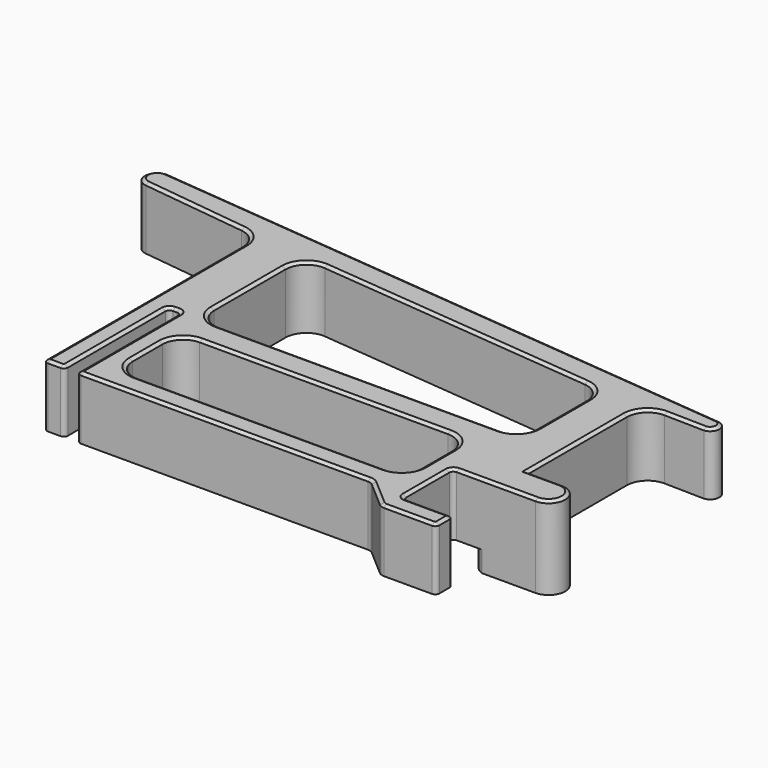
from build123d import *

# Parameters (mm, degrees)
F1_DEPTH      = 19.05
F2_T1_DEPTH   = 75.2234896329
F2_T3_DEPTH   = 3.81
F2_T5_DEPTH   = 37.3962257746
F2_T7_DEPTH   = 1.27
F2_T9_DEPTH   = 88.0190491883
F2_T11_DEPTH  = 10.8349024574
F2_T13_DEPTH  = 14.7622946385
F2_T15_DEPTH  = 3.81
F2_T17_DEPTH  = 12.6952033794
F2_T19_DEPTH  = 16.5052033794
F2_T21_DEPTH  = 24.13
F2_T23_DEPTH  = 10.16
F2_T25_DEPTH  = 35.52184429
F2_T28_ANGLE  = 83.061791683
F2_T30_ANGLE  = 90
F2_T32_ANGLE  = 90
F2_T34_ANGLE  = 90
F2_T36_ANGLE  = 90
F2_T38_ANGLE  = 90
F2_T40_ANGLE  = 40.847550521
F2_T42_ANGLE  = 40.8475505209
F2_T44_ANGLE  = 90
F2_T46_ANGLE  = 90
F2_T48_ANGLE  = 90
F2_T50_ANGLE  = 90
F2_T52_ANGLE  = 180
F2_T53_DEPTH  = 15.1008716715
F2_T58_DEPTH  = 41.6145620658
F2_T63_DEPTH  = 41.6145620658
F2_T69_DEPTH  = 41.6145620658
F2_T73_ANGLE  = 91.1976782387
F2_T74_DEPTH  = 183.8355440501
F2_T77_ANGLE  = 180.467792794
F2_T79_ANGLE  = 176.997776884
F2_T80_DEPTH  = 76.2
F2_T82_DEPTH  = 11.4254270077
F2_T85_ANGLE  = 90
F2_T87_ANGLE  = 90
F2_T89_ANGLE  = 90
F2_T91_ANGLE  = 90
F2_T92_DEPTH  = 19.192433885
F2_T94_DEPTH  = 86.36
F2_T96_DEPTH  = 27.4006934119
F2_T98_DEPTH  = 86.7492082065
F2_T101_ANGLE = 84.5705182986
F2_T103_ANGLE = 90
F2_T105_ANGLE = 90
F2_T107_ANGLE = 95.4294817014
F4_DEPTH      = 6.35


# Not quite as in the source:
# - a fillet or chamfer that OpenCascade refuses, or shapes differently, is made with other operations: its cross-section is extruded or revolved along the edge and cut away or added


with BuildPart() as f1:
    # F0 (on Top) → F1 (new body)
    with BuildSketch(Plane.XY):
        with BuildLine():
            Line((-61.3219774175, -39.9362257746), (-47.7384642892, -39.9362257746))
            Line((-47.7384642892, -39.9362257746), (26.6970717708, -39.9362257746))
            ThreePointArc((26.6970717708, -39.9362257746), (27.5834325804, -40.0958971176), (28.3583552632, -40.5548363924))
            Line((28.3583552632, -40.5548363924), (36.5544444517, -47.6413893822))
            ThreePointArc((36.5544444517, -47.6413893822), (37.3293671345, -48.100328657), (38.215727944, -48.26))
            Line((38.215727944, -48.26), (52.9780225825, -48.26))
            ThreePointArc((52.9780225825, -48.26), (53.8760481946, -47.8880256121), (54.2480225825, -46.99))
            Line((54.2480225825, -46.99), (54.2480225825, -43.18))
            ThreePointArc((54.2480225825, -43.18), (53.8760481946, -42.2819743879), (52.9780225825, -41.91))
            Line((52.9780225825, -41.91), (40.2828192031, -41.91))
            ThreePointArc((40.2828192031, -41.91), (39.3814018681, -41.5366207145), (39.0080225825, -40.6352033794))
            Line((39.0080225825, -40.6352033794), (39.0080225825, -24.13))
            ThreePointArc((39.0080225825, -24.13), (39.3799969704, -23.2319743879), (40.2780225825, -22.86))
            Line((40.2780225825, -22.86), (56.7928192031, -22.86))
            Line((56.7928192031, -22.86), (64.4080225825, -22.86))
            ThreePointArc((64.4080225825, -22.86), (69.4880225825, -17.78), (64.4080225825, -12.7))
            Line((64.4080225825, -12.7), (54.2480225825, -12.7))
            Line((54.2480225825, -12.7), (54.2480225825, 0))
            Line((54.2480225825, 0), (54.2480225825, 24.9692976817))
            ThreePointArc((54.2480225825, 24.9692976817), (56.1550684482, 29.5061091787), (60.730749688, 31.3179104053))
            Line((60.730749688, 31.3179104053), (72.9835318038, 31.0617479373))
            ThreePointArc((72.9835318038, 31.0617479373), (75.4911679584, 33.8910968404), (72.9375934671, 36.6790551646))
            Line((72.9375934671, 36.6790551646), (-110.0535898834, 54.2783185637))
            ThreePointArc((-110.0535898834, 54.2783185637), (-114.147959014, 50.9024071856), (-110.772047636, 46.808038055))
            Line((-110.772047636, 46.808038055), (-78.3349047634, 42.8607628504))
            ThreePointArc((-78.3349047634, 42.8607628504), (-74.3483781836, 40.7674650795), (-72.7519774175, 36.5572638583))
            Line((-72.7519774175, 36.5572638583), (-72.7519774175, 0))
            Line((-72.7519774175, 0), (-72.7519774175, -24.13))
            Line((-72.7519774175, -24.13), (-72.7519774175, -38.6662257746))
            ThreePointArc((-72.7519774175, -38.6662257746), (-72.3800030296, -39.5642513867), (-71.4819774175, -39.9362257746))
            Line((-71.4819774175, -39.9362257746), (-67.6719774175, -39.9362257746))
            ThreePointArc((-67.6719774175, -39.9362257746), (-66.7739518054, -39.5642513867), (-66.4019774175, -38.6662257746))
            Line((-66.4019774175, -38.6662257746), (-66.4019774175, -24.13))
            Line((-66.4019774175, -24.13), (-66.4019774175, -1.27))
            ThreePointArc((-66.4019774175, -1.27), (-66.0300030296, -0.3719743879), (-65.1319774175, 0))
            Line((-65.1319774175, 0), (-63.8619774175, 0))
            ThreePointArc((-63.8619774175, 0), (-62.9639518054, -0.3719743879), (-62.5919774175, -1.27))
            Line((-62.5919774175, -1.27), (-62.5919774175, -24.13))
            Line((-62.5919774175, -24.13), (-62.5919774175, -38.6662257746))
            ThreePointArc((-62.5919774175, -38.6662257746), (-62.2200030296, -39.5642513867), (-61.3219774175, -39.9362257746))
        make_face()
        with BuildLine():
            ThreePointArc((-56.2419774175, -15.0875305593), (-54.382105478, -10.5974024988), (-49.8919774175, -8.7375305593))
            Line((-49.8919774175, -8.7375305593), (26.3080225825, -8.7375305593))
            ThreePointArc((26.3080225825, -8.7375305593), (30.7981506431, -10.5974024988), (32.6580225825, -15.0875305593))
            Line((32.6580225825, -15.0875305593), (32.6580225825, -26.512957567))
            ThreePointArc((32.6580225825, -26.512957567), (30.7981506431, -31.0030856275), (26.3080225825, -32.862957567))
            Line((26.3080225825, -32.862957567), (-49.8919774175, -32.862957567))
            ThreePointArc((-49.8919774175, -32.862957567), (-54.382105478, -31.0030856275), (-56.2419774175, -26.512957567))
            Line((-56.2419774175, -26.512957567), (-56.2419774175, -15.0875305593))
        make_face(mode=Mode.SUBTRACT)
        with BuildLine():
            ThreePointArc((35.798863202, 31.8639440329), (39.8957793841, 29.8148548653), (41.5480225825, 25.542433885))
            Line((41.5480225825, 25.542433885), (41.5480225825, 6.35))
            ThreePointArc((41.5480225825, 6.35), (39.6881506431, 1.8598719395), (35.1980225825, 0))
            Line((35.1980225825, 0), (-51.1619774175, 0))
            ThreePointArc((-51.1619774175, 0), (-55.652105478, 1.8598719395), (-57.5119774175, 6.35))
            Line((-57.5119774175, 6.35), (-57.5119774175, 33.7506934119))
            ThreePointArc((-57.5119774175, 33.7506934119), (-55.4343983978, 38.4484502135), (-50.561136798, 40.0722035598))
            Line((-50.561136798, 40.0722035598), (35.798863202, 31.8639440329))
        make_face(mode=Mode.SUBTRACT)
    extrude(amount=F1_DEPTH)

    # F2: chamfer of 0.635 x 1.0998522628 on 49 edges, made by hand

    # F2_s2 → F2_t1 (cut)
    with BuildSketch(Plane.XZ.offset(-36.5572638583)):
        with BuildLine():
            Line((-71.6140251547, 19.0719970453), (-72.7900774175, 18.3930029547))
            Line((-72.7900774175, 18.3930029547), (-72.8120744627, 18.3930029547))
            ThreePointArc((-72.8120744627, 18.3930029547), (-72.7739744627, 18.7215014774), (-72.7739744627, 19.05))
            Line((-72.7739744627, 19.05), (-72.7519774175, 19.0719970453))
            ThreePointArc((-72.7519774175, 19.0719970453), (-72.1830012861, 19.0719970453), (-71.6140251547, 19.0939940905))
            Line((-71.6140251547, 19.0939940905), (-71.6140251547, 19.0719970453))
        make_face()
    extrude(amount=F2_T1_DEPTH, mode=Mode.SUBTRACT)

    # F2_s4 → F2_t3 (cut)
    with BuildSketch(Plane.YZ.offset(-71.4819774175)):
        with BuildLine():
            Line((-38.7982735118, 19.0719970453), (-39.9743257746, 18.3930029547))
            Line((-39.9743257746, 18.3930029547), (-39.9963228198, 18.3930029547))
            ThreePointArc((-39.9963228198, 18.3930029547), (-39.9582228198, 18.7215014774), (-39.9582228198, 19.05))
            Line((-39.9582228198, 19.05), (-39.9362257746, 19.0719970453))
            ThreePointArc((-39.9362257746, 19.0719970453), (-39.3672496432, 19.0719970453), (-38.7982735118, 19.0939940905))
            Line((-38.7982735118, 19.0939940905), (-38.7982735118, 19.0719970453))
        make_face()
    extrude(amount=F2_T3_DEPTH, mode=Mode.SUBTRACT)

    # F2_s6 → F2_t5 (cut)
    with BuildSketch(Plane.XZ.offset(1.27)):
        with BuildLine():
            Line((-67.5399296803, 19.0719970453), (-66.3638774175, 18.3930029547))
            Line((-66.3638774175, 18.3930029547), (-66.3418803722, 18.3930029547))
            ThreePointArc((-66.3418803722, 18.3930029547), (-66.3799803722, 18.7215014774), (-66.3799803722, 19.05))
            Line((-66.3799803722, 19.05), (-66.4019774175, 19.0719970453))
            ThreePointArc((-66.4019774175, 19.0719970453), (-66.9709535489, 19.0719970453), (-67.5399296803, 19.0939940905))
            Line((-67.5399296803, 19.0939940905), (-67.5399296803, 19.0719970453))
        make_face()
        with BuildLine():
            Line((-61.4540251547, 19.0719970453), (-62.6300774175, 18.3930029547))
            Line((-62.6300774175, 18.3930029547), (-62.6520744627, 18.3930029547))
            ThreePointArc((-62.6520744627, 18.3930029547), (-62.6139744627, 18.7215014774), (-62.6139744627, 19.05))
            Line((-62.6139744627, 19.05), (-62.5919774175, 19.0719970453))
            ThreePointArc((-62.5919774175, 19.0719970453), (-62.0230012861, 19.0719970453), (-61.4540251547, 19.0939940905))
            Line((-61.4540251547, 19.0939940905), (-61.4540251547, 19.0719970453))
        make_face()
    extrude(amount=F2_T5_DEPTH, mode=Mode.SUBTRACT)

    # F2_s8 → F2_t7 (cut)
    with BuildSketch(Plane.YZ.offset(-65.1319774175)):
        with BuildLine():
            Line((1.1379522628, 19.0719970453), (-0.0381, 18.3930029547))
            Line((-0.0381, 18.3930029547), (-0.0600970453, 18.3930029547))
            ThreePointArc((-0.0600970453, 18.3930029547), (-0.0219970453, 18.7215014774), (-0.0219970453, 19.05))
            Line((-0.0219970453, 19.05), (0, 19.0719970453))
            ThreePointArc((0, 19.0719970453), (0.5689761314, 19.0719970453), (1.1379522628, 19.0939940905))
            Line((1.1379522628, 19.0939940905), (1.1379522628, 19.0719970453))
        make_face()
    extrude(amount=F2_T7_DEPTH, mode=Mode.SUBTRACT)

    # F2_s10 → F2_t9 (cut)
    with BuildSketch(Plane.YZ.offset(-61.3219774175)):
        with BuildLine():
            Line((-38.7982735118, 19.0719970453), (-39.9743257746, 18.3930029547))
            Line((-39.9743257746, 18.3930029547), (-39.9963228198, 18.3930029547))
            ThreePointArc((-39.9963228198, 18.3930029547), (-39.9582228198, 18.7215014774), (-39.9582228198, 19.05))
            Line((-39.9582228198, 19.05), (-39.9362257746, 19.0719970453))
            ThreePointArc((-39.9362257746, 19.0719970453), (-39.3672496432, 19.0719970453), (-38.7982735118, 19.0939940905))
            Line((-38.7982735118, 19.0939940905), (-38.7982735118, 19.0719970453))
        make_face()
    extrude(amount=F2_T9_DEPTH, mode=Mode.SUBTRACT)

    # F2_s12 → F2_t11 (cut)
    with BuildSketch(Plane(origin=(36.2920073891, -31.379018402, 0), x_dir=(0, 0, 1), z_dir=(0.7564525127, -0.654048619, 0))):
        with BuildLine():
            Line((19.0719970453, 10.9921125288), (18.3930029547, 12.1681647916))
            Line((18.3930029547, 12.1681647916), (18.3930029547, 12.1901618368))
            ThreePointArc((18.3930029547, 12.1901618368), (18.7215014774, 12.1520618368), (19.05, 12.1520618368))
            Line((19.05, 12.1520618368), (19.0719970453, 12.1300647916))
            ThreePointArc((19.0719970453, 12.1300647916), (19.0719970453, 11.5610886602), (19.0939940905, 10.9921125288))
            Line((19.0939940905, 10.9921125288), (19.0719970453, 10.9921125288))
        make_face()
    extrude(amount=F2_T11_DEPTH, mode=Mode.SUBTRACT)

    # F2_s14 → F2_t13 (cut)
    with BuildSketch(Plane.YZ.offset(38.215727944)):
        with BuildLine():
            Line((-47.1220477372, 19.0719970453), (-48.2981, 18.3930029547))
            Line((-48.2981, 18.3930029547), (-48.3200970453, 18.3930029547))
            ThreePointArc((-48.3200970453, 18.3930029547), (-48.2819970453, 18.7215014774), (-48.2819970453, 19.05))
            Line((-48.2819970453, 19.05), (-48.26, 19.0719970453))
            ThreePointArc((-48.26, 19.0719970453), (-47.6910238686, 19.0719970453), (-47.1220477372, 19.0939940905))
            Line((-47.1220477372, 19.0939940905), (-47.1220477372, 19.0719970453))
        make_face()
    extrude(amount=F2_T13_DEPTH, mode=Mode.SUBTRACT)

    # F2_s16 → F2_t15 (cut)
    with BuildSketch(Plane.XZ.offset(43.18)):
        with BuildLine():
            Line((53.1100703197, 19.0719970453), (54.2861225825, 18.3930029547))
            Line((54.2861225825, 18.3930029547), (54.3081196278, 18.3930029547))
            ThreePointArc((54.3081196278, 18.3930029547), (54.2700196278, 18.7215014774), (54.2700196278, 19.05))
            Line((54.2700196278, 19.05), (54.2480225825, 19.0719970453))
            ThreePointArc((54.2480225825, 19.0719970453), (53.6790464511, 19.0719970453), (53.1100703197, 19.0939940905))
            Line((53.1100703197, 19.0939940905), (53.1100703197, 19.0719970453))
        make_face()
    extrude(amount=F2_T15_DEPTH, mode=Mode.SUBTRACT)

    # F2_s18 → F2_t17 (cut)
    with BuildSketch(Plane.YZ.offset(40.2828192031)):
        with BuildLine():
            Line((-43.0479522628, 19.0719970453), (-41.8719, 18.3930029547))
            Line((-41.8719, 18.3930029547), (-41.8499029547, 18.3930029547))
            ThreePointArc((-41.8499029547, 18.3930029547), (-41.8880029547, 18.7215014774), (-41.8880029547, 19.05))
            Line((-41.8880029547, 19.05), (-41.91, 19.0719970453))
            ThreePointArc((-41.91, 19.0719970453), (-42.4789761314, 19.0719970453), (-43.0479522628, 19.0939940905))
            Line((-43.0479522628, 19.0939940905), (-43.0479522628, 19.0719970453))
        make_face()
    extrude(amount=F2_T17_DEPTH, mode=Mode.SUBTRACT)

    # F2_s20 → F2_t19 (cut)
    with BuildSketch(Plane.XZ.offset(24.13)):
        with BuildLine():
            Line((37.8700703197, 19.0719970453), (39.0461225825, 18.3930029547))
            Line((39.0461225825, 18.3930029547), (39.0681196278, 18.3930029547))
            ThreePointArc((39.0681196278, 18.3930029547), (39.0300196278, 18.7215014774), (39.0300196278, 19.05))
            Line((39.0300196278, 19.05), (39.0080225825, 19.0719970453))
            ThreePointArc((39.0080225825, 19.0719970453), (38.4390464511, 19.0719970453), (37.8700703197, 19.0939940905))
            Line((37.8700703197, 19.0939940905), (37.8700703197, 19.0719970453))
        make_face()
    extrude(amount=F2_T19_DEPTH, mode=Mode.SUBTRACT)

    # F2_s22 → F2_t21 (cut)
    with BuildSketch(Plane.YZ.offset(40.2780225825)):
        with BuildLine():
            Line((-21.7220477372, 19.0719970453), (-22.8981, 18.3930029547))
            Line((-22.8981, 18.3930029547), (-22.9200970453, 18.3930029547))
            ThreePointArc((-22.9200970453, 18.3930029547), (-22.8819970453, 18.7215014774), (-22.8819970453, 19.05))
            Line((-22.8819970453, 19.05), (-22.86, 19.0719970453))
            ThreePointArc((-22.86, 19.0719970453), (-22.2910238686, 19.0719970453), (-21.7220477372, 19.0939940905))
            Line((-21.7220477372, 19.0939940905), (-21.7220477372, 19.0719970453))
        make_face()
    extrude(amount=F2_T21_DEPTH, mode=Mode.SUBTRACT)

    # F2_s24 → F2_t23 (cut)
    with BuildSketch(Plane.YZ.offset(54.2480225825)):
        with BuildLine():
            Line((-13.8379522628, 19.0719970453), (-12.6619, 18.3930029547))
            Line((-12.6619, 18.3930029547), (-12.6399029547, 18.3930029547))
            ThreePointArc((-12.6399029547, 18.3930029547), (-12.6780029547, 18.7215014774), (-12.6780029547, 19.05))
            Line((-12.6780029547, 19.05), (-12.7, 19.0719970453))
            ThreePointArc((-12.7, 19.0719970453), (-13.2689761314, 19.0719970453), (-13.8379522628, 19.0939940905))
            Line((-13.8379522628, 19.0939940905), (-13.8379522628, 19.0719970453))
        make_face()
    extrude(amount=F2_T23_DEPTH, mode=Mode.SUBTRACT)

    # F2_s26 → F2_t25 (cut)
    with BuildSketch(Plane(origin=(-117.5931471997, 14.3099075031, 0), x_dir=(0, 0, 1), z_dir=(0.9926770066, -0.1207988432, 0))):
        with BuildLine():
            Line((19.0719970453, -34.2220801565), (18.3930029547, -33.0460278937))
            Line((18.3930029547, -33.0460278937), (18.3930029547, -33.0240308484))
            ThreePointArc((18.3930029547, -33.0240308484), (18.7215014774, -33.0621308484), (19.05, -33.0621308484))
            Line((19.05, -33.0621308484), (19.0719970453, -33.0841278937))
            ThreePointArc((19.0719970453, -33.0841278937), (19.0719970453, -33.6531040251), (19.0939940905, -34.2220801565))
            Line((19.0939940905, -34.2220801565), (19.0719970453, -34.2220801565))
        make_face()
    extrude(amount=F2_T25_DEPTH, mode=Mode.SUBTRACT)

    # F2_s27 → F2_t28 (revolve, cut)
    with BuildSketch(Plane(origin=(-82.3314291399, 10.0189098059, 0), x_dir=(0, 0, 1), z_dir=(-0.9926770066, 0.1207988432, 0))):
        with BuildLine():
            Line((18.3930029547, 33.0460278937), (19.0719970453, 34.2220801565))
            Line((19.0719970453, 34.2220801565), (19.0939940905, 34.2220801565))
            ThreePointArc((19.0939940905, 34.2220801565), (19.0719970453, 33.6531040251), (19.0719970453, 33.0841278937))
            Line((19.0719970453, 33.0841278937), (19.05, 33.0621308484))
            ThreePointArc((19.05, 33.0621308484), (18.7215014774, 33.0621308484), (18.3930029547, 33.0240308484))
            Line((18.3930029547, 33.0240308484), (18.3930029547, 33.0460278937))
        make_face()
    revolve(axis=Axis((-79.1019774175, 36.5572638583, 19.05), (0, 0, -1)), revolution_arc=F2_T28_ANGLE, mode=Mode.SUBTRACT)

    # F2_s29 → F2_t30 (revolve, cut)
    with BuildSketch(Plane.XZ.offset(38.6662257746)):
        with BuildLine():
            Line((-71.6140251547, 19.0719970453), (-72.7900774175, 18.3930029547))
            Line((-72.7900774175, 18.3930029547), (-72.8120744627, 18.3930029547))
            ThreePointArc((-72.8120744627, 18.3930029547), (-72.7739744627, 18.7215014774), (-72.7739744627, 19.05))
            Line((-72.7739744627, 19.05), (-72.7519774175, 19.0719970453))
            ThreePointArc((-72.7519774175, 19.0719970453), (-72.1830012861, 19.0719970453), (-71.6140251547, 19.0939940905))
            Line((-71.6140251547, 19.0939940905), (-71.6140251547, 19.0719970453))
        make_face()
    revolve(axis=Axis((-71.4819774175, -38.6662257746, 19.05), (0, 0, 1)), revolution_arc=F2_T30_ANGLE, mode=Mode.SUBTRACT)

    # F2_s31 → F2_t32 (revolve, cut)
    with BuildSketch(Plane.YZ.offset(-67.6719774175)):
        with BuildLine():
            Line((-38.7982735118, 19.0719970453), (-39.9743257746, 18.3930029547))
            Line((-39.9743257746, 18.3930029547), (-39.9963228198, 18.3930029547))
            ThreePointArc((-39.9963228198, 18.3930029547), (-39.9582228198, 18.7215014774), (-39.9582228198, 19.05))
            Line((-39.9582228198, 19.05), (-39.9362257746, 19.0719970453))
            ThreePointArc((-39.9362257746, 19.0719970453), (-39.3672496432, 19.0719970453), (-38.7982735118, 19.0939940905))
            Line((-38.7982735118, 19.0939940905), (-38.7982735118, 19.0719970453))
        make_face()
    revolve(axis=Axis((-67.6719774175, -38.6662257746, 19.05), (0, 0, 1)), revolution_arc=F2_T32_ANGLE, mode=Mode.SUBTRACT)

    # F2_s33 → F2_t34 (revolve, cut)
    with BuildSketch(Plane.XZ.offset(1.27)):
        with BuildLine():
            Line((-67.5399296803, 19.0719970453), (-66.3638774175, 18.3930029547))
            Line((-66.3638774175, 18.3930029547), (-66.3418803722, 18.3930029547))
            ThreePointArc((-66.3418803722, 18.3930029547), (-66.3799803722, 18.7215014774), (-66.3799803722, 19.05))
            Line((-66.3799803722, 19.05), (-66.4019774175, 19.0719970453))
            ThreePointArc((-66.4019774175, 19.0719970453), (-66.9709535489, 19.0719970453), (-67.5399296803, 19.0939940905))
            Line((-67.5399296803, 19.0939940905), (-67.5399296803, 19.0719970453))
        make_face()
    revolve(axis=Axis((-65.1319774175, -1.27, 19.05), (0, 0, -1)), revolution_arc=F2_T34_ANGLE, mode=Mode.SUBTRACT)

    # F2_s35 → F2_t36 (revolve, cut)
    with BuildSketch(Plane.YZ.offset(-63.8619774175)):
        with BuildLine():
            Line((1.1379522628, 19.0719970453), (-0.0381, 18.3930029547))
            Line((-0.0381, 18.3930029547), (-0.0600970453, 18.3930029547))
            ThreePointArc((-0.0600970453, 18.3930029547), (-0.0219970453, 18.7215014774), (-0.0219970453, 19.05))
            Line((-0.0219970453, 19.05), (0, 19.0719970453))
            ThreePointArc((0, 19.0719970453), (0.5689761314, 19.0719970453), (1.1379522628, 19.0939940905))
            Line((1.1379522628, 19.0939940905), (1.1379522628, 19.0719970453))
        make_face()
    revolve(axis=Axis((-63.8619774175, -1.27, 19.05), (0, 0, -1)), revolution_arc=F2_T36_ANGLE, mode=Mode.SUBTRACT)

    # F2_s37 → F2_t38 (revolve, cut)
    with BuildSketch(Plane.XZ.offset(38.6662257746)):
        with BuildLine():
            Line((-61.4540251547, 19.0719970453), (-62.6300774175, 18.3930029547))
            Line((-62.6300774175, 18.3930029547), (-62.6520744627, 18.3930029547))
            ThreePointArc((-62.6520744627, 18.3930029547), (-62.6139744627, 18.7215014774), (-62.6139744627, 19.05))
            Line((-62.6139744627, 19.05), (-62.5919774175, 19.0719970453))
            ThreePointArc((-62.5919774175, 19.0719970453), (-62.0230012861, 19.0719970453), (-61.4540251547, 19.0939940905))
            Line((-61.4540251547, 19.0939940905), (-61.4540251547, 19.0719970453))
        make_face()
    revolve(axis=Axis((-61.3219774175, -38.6662257746, 19.05), (0, 0, 1)), revolution_arc=F2_T38_ANGLE, mode=Mode.SUBTRACT)

    # F2_s39 → F2_t40 (revolve, cut)
    with BuildSketch(Plane.YZ.offset(26.6970717708)):
        with BuildLine():
            Line((-38.7982735118, 19.0719970453), (-39.9743257746, 18.3930029547))
            Line((-39.9743257746, 18.3930029547), (-39.9963228198, 18.3930029547))
            ThreePointArc((-39.9963228198, 18.3930029547), (-39.9582228198, 18.7215014774), (-39.9582228198, 19.05))
            Line((-39.9582228198, 19.05), (-39.9362257746, 19.0719970453))
            ThreePointArc((-39.9362257746, 19.0719970453), (-39.3672496432, 19.0719970453), (-38.7982735118, 19.0939940905))
            Line((-38.7982735118, 19.0939940905), (-38.7982735118, 19.0719970453))
        make_face()
    revolve(axis=Axis((26.6970717708, -42.4762257746, 19.05), (0, 0, -1)), revolution_arc=F2_T40_ANGLE, mode=Mode.SUBTRACT)

    # F2_s41 → F2_t42 (revolve, cut)
    with BuildSketch(Plane(origin=(44.4880965775, -38.4655713918, 0), x_dir=(0, 0, 1), z_dir=(-0.7564525127, 0.654048619, 0))):
        with BuildLine():
            Line((19.0719970453, -10.9921125288), (18.3930029547, -12.1681647916))
            Line((18.3930029547, -12.1681647916), (18.3930029547, -12.1901618368))
            ThreePointArc((18.3930029547, -12.1901618368), (18.7215014774, -12.1520618368), (19.05, -12.1520618368))
            Line((19.05, -12.1520618368), (19.0719970453, -12.1300647916))
            ThreePointArc((19.0719970453, -12.1300647916), (19.0719970453, -11.5610886602), (19.0939940905, -10.9921125288))
            Line((19.0939940905, -10.9921125288), (19.0719970453, -10.9921125288))
        make_face()
    revolve(axis=Axis((38.215727944, -45.72, 19.05), (0, 0, 1)), revolution_arc=F2_T42_ANGLE, mode=Mode.SUBTRACT)

    # F2_s43 → F2_t44 (revolve, cut)
    with BuildSketch(Plane.YZ.offset(52.9780225825)):
        with BuildLine():
            Line((-47.1220477372, 19.0719970453), (-48.2981, 18.3930029547))
            Line((-48.2981, 18.3930029547), (-48.3200970453, 18.3930029547))
            ThreePointArc((-48.3200970453, 18.3930029547), (-48.2819970453, 18.7215014774), (-48.2819970453, 19.05))
            Line((-48.2819970453, 19.05), (-48.26, 19.0719970453))
            ThreePointArc((-48.26, 19.0719970453), (-47.6910238686, 19.0719970453), (-47.1220477372, 19.0939940905))
            Line((-47.1220477372, 19.0939940905), (-47.1220477372, 19.0719970453))
        make_face()
    revolve(axis=Axis((52.9780225825, -46.99, 19.05), (0, 0, 1)), revolution_arc=F2_T44_ANGLE, mode=Mode.SUBTRACT)

    # F2_s45 → F2_t46 (revolve, cut)
    with BuildSketch(Plane.XZ.offset(43.18)):
        with BuildLine():
            Line((53.1100703197, 19.0719970453), (54.2861225825, 18.3930029547))
            Line((54.2861225825, 18.3930029547), (54.3081196278, 18.3930029547))
            ThreePointArc((54.3081196278, 18.3930029547), (54.2700196278, 18.7215014774), (54.2700196278, 19.05))
            Line((54.2700196278, 19.05), (54.2480225825, 19.0719970453))
            ThreePointArc((54.2480225825, 19.0719970453), (53.6790464511, 19.0719970453), (53.1100703197, 19.0939940905))
            Line((53.1100703197, 19.0939940905), (53.1100703197, 19.0719970453))
        make_face()
    revolve(axis=Axis((52.9780225825, -43.18, 19.05), (0, 0, 1)), revolution_arc=F2_T46_ANGLE, mode=Mode.SUBTRACT)

    # F2_s47 → F2_t48 (revolve, cut)
    with BuildSketch(Plane.YZ.offset(40.2828192031)):
        with BuildLine():
            Line((-43.0479522628, 19.0719970453), (-41.8719, 18.3930029547))
            Line((-41.8719, 18.3930029547), (-41.8499029547, 18.3930029547))
            ThreePointArc((-41.8499029547, 18.3930029547), (-41.8880029547, 18.7215014774), (-41.8880029547, 19.05))
            Line((-41.8880029547, 19.05), (-41.91, 19.0719970453))
            ThreePointArc((-41.91, 19.0719970453), (-42.4789761314, 19.0719970453), (-43.0479522628, 19.0939940905))
            Line((-43.0479522628, 19.0939940905), (-43.0479522628, 19.0719970453))
        make_face()
    revolve(axis=Axis((40.2828192031, -40.6352033794, 19.05), (0, 0, -1)), revolution_arc=F2_T48_ANGLE, mode=Mode.SUBTRACT)

    # F2_s49 → F2_t50 (revolve, cut)
    with BuildSketch(Plane.XZ.offset(24.13)):
        with BuildLine():
            Line((37.8700703197, 19.0719970453), (39.0461225825, 18.3930029547))
            Line((39.0461225825, 18.3930029547), (39.0681196278, 18.3930029547))
            ThreePointArc((39.0681196278, 18.3930029547), (39.0300196278, 18.7215014774), (39.0300196278, 19.05))
            Line((39.0300196278, 19.05), (39.0080225825, 19.0719970453))
            ThreePointArc((39.0080225825, 19.0719970453), (38.4390464511, 19.0719970453), (37.8700703197, 19.0939940905))
            Line((37.8700703197, 19.0939940905), (37.8700703197, 19.0719970453))
        make_face()
    revolve(axis=Axis((40.2780225825, -24.13, 19.05), (0, 0, -1)), revolution_arc=F2_T50_ANGLE, mode=Mode.SUBTRACT)

    # F2_s51 → F2_t52 (revolve, cut)
    with BuildSketch(Plane.YZ.offset(64.4080225825)):
        with BuildLine():
            Line((-21.7220477372, 19.0719970453), (-22.8981, 18.3930029547))
            Line((-22.8981, 18.3930029547), (-22.9200970453, 18.3930029547))
            ThreePointArc((-22.9200970453, 18.3930029547), (-22.8819970453, 18.7215014774), (-22.8819970453, 19.05))
            Line((-22.8819970453, 19.05), (-22.86, 19.0719970453))
            ThreePointArc((-22.86, 19.0719970453), (-22.2910238686, 19.0719970453), (-21.7220477372, 19.0939940905))
            Line((-21.7220477372, 19.0939940905), (-21.7220477372, 19.0719970453))
        make_face()
    revolve(axis=Axis((64.4080225825, -17.78, 19.05), (0, 0, 1)), revolution_arc=F2_T52_ANGLE, mode=Mode.SUBTRACT)

    # F2_s54 → F2_t53 (cut)
    with BuildSketch(Plane(origin=(60.049756029, -1.2554286502, 0), x_dir=(0, 0, 1), z_dir=(0.9997815313, -0.0209019064, 0))):
        with BuildLine():
            Line((18.3930029547, -32.5423568659), (19.0719970453, -33.7184091287))
            Line((19.0719970453, -33.7184091287), (19.0939940905, -33.7184091287))
            ThreePointArc((19.0939940905, -33.7184091287), (19.0719970453, -33.1494329973), (19.0719970453, -32.5804568659))
            Line((19.0719970453, -32.5804568659), (19.05, -32.5584598207))
            ThreePointArc((19.05, -32.5584598207), (18.7215014774, -32.5584598207), (18.3930029547, -32.5203598207))
            Line((18.3930029547, -32.5203598207), (18.3930029547, -32.5423568659))
        make_face()
    extrude(amount=F2_T53_DEPTH, mode=Mode.SUBTRACT)


with BuildPart() as f2_tool56:
    # F2_s57 → F2_t58 (new body)
    with BuildSketch(Plane.XZ.offset(-24.9692976817)):
        with BuildLine():
            Line((54.2861225825, 18.3930029547), (53.1100703197, 19.0719970453))
            Line((53.1100703197, 19.0719970453), (53.1100703197, 19.0939940905))
            ThreePointArc((53.1100703197, 19.0939940905), (53.6790464511, 19.0719970453), (54.2480225825, 19.0719970453))
            Line((54.2480225825, 19.0719970453), (54.2700196278, 19.05))
            ThreePointArc((54.2700196278, 19.05), (54.2700196278, 18.7215014774), (54.3081196278, 18.3930029547))
            Line((54.3081196278, 18.3930029547), (54.2861225825, 18.3930029547))
        make_face()
    extrude(amount=F2_T58_DEPTH)

    split(bisect_by=Plane.XZ.offset(12.7), keep=Keep.BOTTOM)


with BuildPart() as f1_1:
    add(f1.part)

    # F2_t55: cut F2_tool56
    add(f2_tool56.part, mode=Mode.SUBTRACT)


with BuildPart() as f2_tool61:
    # F2_s62 → F2_t63 (new body)
    with BuildSketch(Plane.XZ.offset(-24.9692976817)):
        with BuildLine():
            Line((54.2861225825, 18.3930029547), (53.1100703197, 19.0719970453))
            Line((53.1100703197, 19.0719970453), (53.1100703197, 19.0939940905))
            ThreePointArc((53.1100703197, 19.0939940905), (53.6790464511, 19.0719970453), (54.2480225825, 19.0719970453))
            Line((54.2480225825, 19.0719970453), (54.2700196278, 19.05))
            ThreePointArc((54.2700196278, 19.05), (54.2700196278, 18.7215014774), (54.3081196278, 18.3930029547))
            Line((54.3081196278, 18.3930029547), (54.2861225825, 18.3930029547))
        make_face()
    extrude(amount=F2_T63_DEPTH)

    split(bisect_by=Plane.XZ.offset(12.7), keep=Keep.TOP)

    split(bisect_by=Plane(origin=(0, 4.7989289053, 8.311988686), x_dir=(1, 0, 0), z_dir=(0, 0.5, 0.8660254038)), keep=Keep.TOP)


with BuildPart() as f1_2:
    add(f1_1.part)

    # F2_t60: cut F2_tool61
    add(f2_tool61.part, mode=Mode.SUBTRACT)


with BuildPart() as f2_tool67:
    # F2_s68 → F2_t69 (new body)
    with BuildSketch(Plane.XZ.offset(-24.9692976817)):
        with BuildLine():
            Line((54.2861225825, 18.3930029547), (53.1100703197, 19.0719970453))
            Line((53.1100703197, 19.0719970453), (53.1100703197, 19.0939940905))
            ThreePointArc((53.1100703197, 19.0939940905), (53.6790464511, 19.0719970453), (54.2480225825, 19.0719970453))
            Line((54.2480225825, 19.0719970453), (54.2700196278, 19.05))
            ThreePointArc((54.2700196278, 19.05), (54.2700196278, 18.7215014774), (54.3081196278, 18.3930029547))
            Line((54.3081196278, 18.3930029547), (54.2861225825, 18.3930029547))
        make_face()
    extrude(amount=F2_T69_DEPTH)

    split(bisect_by=Plane.XZ.offset(12.7), keep=Keep.BOTTOM)

    split(bisect_by=Plane(origin=(0, 4.7989289053, 8.311988686), x_dir=(1, 0, 0), z_dir=(0, -0.5, -0.8660254038)), keep=Keep.TOP)


with BuildPart() as f1_3:
    add(f1_2.part)

    # F2_t66: cut F2_tool67
    add(f2_tool67.part, mode=Mode.SUBTRACT)

    # F2_s72 → F2_t73 (revolve, cut)
    with BuildSketch(Plane.XZ.offset(-24.9692976817)):
        with BuildLine():
            Line((54.2861225825, 18.3930029547), (53.1100703197, 19.0719970453))
            Line((53.1100703197, 19.0719970453), (53.1100703197, 19.0939940905))
            ThreePointArc((53.1100703197, 19.0939940905), (53.6790464511, 19.0719970453), (54.2480225825, 19.0719970453))
            Line((54.2480225825, 19.0719970453), (54.2700196278, 19.05))
            ThreePointArc((54.2700196278, 19.05), (54.2700196278, 18.7215014774), (54.3081196278, 18.3930029547))
            Line((54.3081196278, 18.3930029547), (54.2861225825, 18.3930029547))
        make_face()
    revolve(axis=Axis((60.5980225825, 24.9692976817, 19.05), (0, 0, -1)), revolution_arc=F2_T73_ANGLE, mode=Mode.SUBTRACT)

    # F2_s75 → F2_t74 (cut)
    with BuildSketch(Plane(origin=(68.7738292713, -6.6143554796, 0), x_dir=(0, 0, 1), z_dir=(-0.995406978, 0.0957337358, 0))):
        with BuildLine():
            Line((18.3930029547, 43.5312757576), (19.0719970453, 42.3552234948))
            Line((19.0719970453, 42.3552234948), (19.0939940905, 42.3552234948))
            ThreePointArc((19.0939940905, 42.3552234948), (19.0719970453, 42.9241996262), (19.0719970453, 43.4931757576))
            Line((19.0719970453, 43.4931757576), (19.05, 43.5151728029))
            ThreePointArc((19.05, 43.5151728029), (18.7215014774, 43.5151728029), (18.3930029547, 43.5532728029))
            Line((18.3930029547, 43.5532728029), (18.3930029547, 43.5312757576))
        make_face()
    extrude(amount=F2_T74_DEPTH, mode=Mode.SUBTRACT)

    # F2_s76 → F2_t77 (revolve, cut)
    with BuildSketch(Plane(origin=(68.3849992898, -7.1409103394, 0), x_dir=(0, 0, 1), z_dir=(-0.9945921898, 0.1038574793, 0))):
        with BuildLine():
            Line((18.3930029547, 38.3697640989), (19.0719970453, 39.5458163617))
            Line((19.0719970453, 39.5458163617), (19.0939940905, 39.5458163617))
            ThreePointArc((19.0939940905, 39.5458163617), (19.0719970453, 38.9768402303), (19.0719970453, 38.4078640989))
            Line((19.0719970453, 38.4078640989), (19.05, 38.3858670537))
            ThreePointArc((19.05, 38.3858670537), (18.7215014774, 38.3858670537), (18.3930029547, 38.3477670537))
            Line((18.3930029547, 38.3477670537), (18.3930029547, 38.3697640989))
        make_face()
    revolve(axis=Axis((72.6672391749, 33.8680027518, 19.05), (0, 0, 1)), revolution_arc=F2_T77_ANGLE, mode=Mode.SUBTRACT)

    # F2_s78 → F2_t79 (revolve, cut)
    with BuildSketch(Plane(origin=(-114.2173540791, 10.9849079195, 0), x_dir=(0, 0, 1), z_dir=(0.995406978, -0.0957337358, 0))):
        with BuildLine():
            Line((18.3930029547, -43.5312757576), (19.0719970453, -42.3552234948))
            Line((19.0719970453, -42.3552234948), (19.0939940905, -42.3552234948))
            ThreePointArc((19.0939940905, -42.3552234948), (19.0719970453, -42.9241996262), (19.0719970453, -43.4931757576))
            Line((19.0719970453, -43.4931757576), (19.05, -43.5151728029))
            ThreePointArc((19.05, -43.5151728029), (18.7215014774, -43.5151728029), (18.3930029547, -43.5532728029))
            Line((18.3930029547, -43.5532728029), (18.3930029547, -43.5312757576))
        make_face()
    revolve(axis=Axis((-110.4128187597, 50.5431783093, 19.05), (0, 0, 1)), revolution_arc=F2_T79_ANGLE, mode=Mode.SUBTRACT)

    # F2_s81 → F2_t80 (cut)
    with BuildSketch(Plane.YZ.offset(-49.8919774175)):
        with BuildLine():
            Line((-8.7756305593, 18.3930029547), (-7.5995782965, 19.0719970453))
            Line((-7.5995782965, 19.0719970453), (-7.5995782965, 19.0939940905))
            ThreePointArc((-7.5995782965, 19.0939940905), (-8.1685544279, 19.0719970453), (-8.7375305593, 19.0719970453))
            Line((-8.7375305593, 19.0719970453), (-8.7595276046, 19.05))
            ThreePointArc((-8.7595276046, 19.05), (-8.7595276046, 18.7215014774), (-8.7976276046, 18.3930029547))
            Line((-8.7976276046, 18.3930029547), (-8.7756305593, 18.3930029547))
        make_face()
        with BuildLine():
            Line((-32.824857567, 18.3930029547), (-34.0009098298, 19.0719970453))
            Line((-34.0009098298, 19.0719970453), (-34.0009098298, 19.0939940905))
            ThreePointArc((-34.0009098298, 19.0939940905), (-33.4319336984, 19.0719970453), (-32.862957567, 19.0719970453))
            Line((-32.862957567, 19.0719970453), (-32.8409605217, 19.05))
            ThreePointArc((-32.8409605217, 19.05), (-32.8409605217, 18.7215014774), (-32.8028605217, 18.3930029547))
            Line((-32.8028605217, 18.3930029547), (-32.824857567, 18.3930029547))
        make_face()
    extrude(amount=F2_T80_DEPTH, mode=Mode.SUBTRACT)

    # F2_s83 → F2_t82 (cut)
    with BuildSketch(Plane.XZ.offset(15.0875305593)):
        with BuildLine():
            Line((32.6199225825, 18.3930029547), (33.7959748453, 19.0719970453))
            Line((33.7959748453, 19.0719970453), (33.7959748453, 19.0939940905))
            ThreePointArc((33.7959748453, 19.0939940905), (33.2269987139, 19.0719970453), (32.6580225825, 19.0719970453))
            Line((32.6580225825, 19.0719970453), (32.6360255373, 19.05))
            ThreePointArc((32.6360255373, 19.05), (32.6360255373, 18.7215014774), (32.5979255373, 18.3930029547))
            Line((32.5979255373, 18.3930029547), (32.6199225825, 18.3930029547))
        make_face()
        with BuildLine():
            Line((-56.2038774175, 18.3930029547), (-57.3799296803, 19.0719970453))
            Line((-57.3799296803, 19.0719970453), (-57.3799296803, 19.0939940905))
            ThreePointArc((-57.3799296803, 19.0939940905), (-56.8109535489, 19.0719970453), (-56.2419774175, 19.0719970453))
            Line((-56.2419774175, 19.0719970453), (-56.2199803722, 19.05))
            ThreePointArc((-56.2199803722, 19.05), (-56.2199803722, 18.7215014774), (-56.1818803722, 18.3930029547))
            Line((-56.1818803722, 18.3930029547), (-56.2038774175, 18.3930029547))
        make_face()
    extrude(amount=F2_T82_DEPTH, mode=Mode.SUBTRACT)

    # F2_s84 → F2_t85 (revolve, cut)
    with BuildSketch(Plane.XZ.offset(15.0875305593)):
        with BuildLine():
            Line((-56.2038774175, 18.3930029547), (-57.3799296803, 19.0719970453))
            Line((-57.3799296803, 19.0719970453), (-57.3799296803, 19.0939940905))
            ThreePointArc((-57.3799296803, 19.0939940905), (-56.8109535489, 19.0719970453), (-56.2419774175, 19.0719970453))
            Line((-56.2419774175, 19.0719970453), (-56.2199803722, 19.05))
            ThreePointArc((-56.2199803722, 19.05), (-56.2199803722, 18.7215014774), (-56.1818803722, 18.3930029547))
            Line((-56.1818803722, 18.3930029547), (-56.2038774175, 18.3930029547))
        make_face()
    revolve(axis=Axis((-49.8919774175, -15.0875305593, 19.05), (0, 0, -1)), revolution_arc=F2_T85_ANGLE, mode=Mode.SUBTRACT)

    # F2_s86 → F2_t87 (revolve, cut)
    with BuildSketch(Plane.YZ.offset(26.3080225825)):
        with BuildLine():
            Line((-8.7756305593, 18.3930029547), (-7.5995782965, 19.0719970453))
            Line((-7.5995782965, 19.0719970453), (-7.5995782965, 19.0939940905))
            ThreePointArc((-7.5995782965, 19.0939940905), (-8.1685544279, 19.0719970453), (-8.7375305593, 19.0719970453))
            Line((-8.7375305593, 19.0719970453), (-8.7595276046, 19.05))
            ThreePointArc((-8.7595276046, 19.05), (-8.7595276046, 18.7215014774), (-8.7976276046, 18.3930029547))
            Line((-8.7976276046, 18.3930029547), (-8.7756305593, 18.3930029547))
        make_face()
    revolve(axis=Axis((26.3080225825, -15.0875305593, 19.05), (0, 0, -1)), revolution_arc=F2_T87_ANGLE, mode=Mode.SUBTRACT)

    # F2_s88 → F2_t89 (revolve, cut)
    with BuildSketch(Plane.XZ.offset(26.512957567)):
        with BuildLine():
            Line((32.6199225825, 18.3930029547), (33.7959748453, 19.0719970453))
            Line((33.7959748453, 19.0719970453), (33.7959748453, 19.0939940905))
            ThreePointArc((33.7959748453, 19.0939940905), (33.2269987139, 19.0719970453), (32.6580225825, 19.0719970453))
            Line((32.6580225825, 19.0719970453), (32.6360255373, 19.05))
            ThreePointArc((32.6360255373, 19.05), (32.6360255373, 18.7215014774), (32.5979255373, 18.3930029547))
            Line((32.5979255373, 18.3930029547), (32.6199225825, 18.3930029547))
        make_face()
    revolve(axis=Axis((26.3080225825, -26.512957567, 19.05), (0, 0, -1)), revolution_arc=F2_T89_ANGLE, mode=Mode.SUBTRACT)

    # F2_s90 → F2_t91 (revolve, cut)
    with BuildSketch(Plane.YZ.offset(-49.8919774175)):
        with BuildLine():
            Line((-32.824857567, 18.3930029547), (-34.0009098298, 19.0719970453))
            Line((-34.0009098298, 19.0719970453), (-34.0009098298, 19.0939940905))
            ThreePointArc((-34.0009098298, 19.0939940905), (-33.4319336984, 19.0719970453), (-32.862957567, 19.0719970453))
            Line((-32.862957567, 19.0719970453), (-32.8409605217, 19.05))
            ThreePointArc((-32.8409605217, 19.05), (-32.8409605217, 18.7215014774), (-32.8028605217, 18.3930029547))
            Line((-32.8028605217, 18.3930029547), (-32.824857567, 18.3930029547))
        make_face()
    revolve(axis=Axis((-49.8919774175, -26.512957567, 19.05), (0, 0, -1)), revolution_arc=F2_T91_ANGLE, mode=Mode.SUBTRACT)

    # F2_s93 → F2_t92 (cut)
    with BuildSketch(Plane.XZ.offset(-25.542433885)):
        with BuildLine():
            Line((41.5099225825, 18.3930029547), (42.6859748453, 19.0719970453))
            Line((42.6859748453, 19.0719970453), (42.6859748453, 19.0939940905))
            ThreePointArc((42.6859748453, 19.0939940905), (42.1169987139, 19.0719970453), (41.5480225825, 19.0719970453))
            Line((41.5480225825, 19.0719970453), (41.5260255373, 19.05))
            ThreePointArc((41.5260255373, 19.05), (41.5260255373, 18.7215014774), (41.4879255373, 18.3930029547))
            Line((41.4879255373, 18.3930029547), (41.5099225825, 18.3930029547))
        make_face()
    extrude(amount=F2_T92_DEPTH, mode=Mode.SUBTRACT)

    # F2_s95 → F2_t94 (cut)
    with BuildSketch(Plane.YZ.offset(-51.1619774175)):
        with BuildLine():
            Line((0.0381, 18.3930029547), (-1.1379522628, 19.0719970453))
            Line((-1.1379522628, 19.0719970453), (-1.1379522628, 19.0939940905))
            ThreePointArc((-1.1379522628, 19.0939940905), (-0.5689761314, 19.0719970453), (0, 19.0719970453))
            Line((0, 19.0719970453), (0.0219970453, 19.05))
            ThreePointArc((0.0219970453, 19.05), (0.0219970453, 18.7215014774), (0.0600970453, 18.3930029547))
            Line((0.0600970453, 18.3930029547), (0.0381, 18.3930029547))
        make_face()
    extrude(amount=F2_T94_DEPTH, mode=Mode.SUBTRACT)

    # F2_s97 → F2_t96 (cut)
    with BuildSketch(Plane.XZ.offset(-33.7506934119)):
        with BuildLine():
            Line((-57.4738774175, 18.3930029547), (-58.6499296803, 19.0719970453))
            Line((-58.6499296803, 19.0719970453), (-58.6499296803, 19.0939940905))
            ThreePointArc((-58.6499296803, 19.0939940905), (-58.0809535489, 19.0719970453), (-57.5119774175, 19.0719970453))
            Line((-57.5119774175, 19.0719970453), (-57.4899803722, 19.05))
            ThreePointArc((-57.4899803722, 19.05), (-57.4899803722, 18.7215014774), (-57.4518803722, 18.3930029547))
            Line((-57.4518803722, 18.3930029547), (-57.4738774175, 18.3930029547))
        make_face()
    extrude(amount=F2_T96_DEPTH, mode=Mode.SUBTRACT)

    # F2_s99 → F2_t98 (cut)
    with BuildSketch(Plane(origin=(-53.8831034358, 5.121427711, 0), x_dir=(0, 0, 1), z_dir=(0.9955134091, -0.09462057, 0))):
        with BuildLine():
            Line((18.3930029547, -35.0701923934), (19.0719970453, -36.2462446562))
            Line((19.0719970453, -36.2462446562), (19.0939940905, -36.2462446562))
            ThreePointArc((19.0939940905, -36.2462446562), (19.0719970453, -35.6772685248), (19.0719970453, -35.1082923934))
            Line((19.0719970453, -35.1082923934), (19.05, -35.0862953481))
            ThreePointArc((19.05, -35.0862953481), (18.7215014774, -35.0862953481), (18.3930029547, -35.0481953481))
            Line((18.3930029547, -35.0481953481), (18.3930029547, -35.0701923934))
        make_face()
    extrude(amount=F2_T98_DEPTH, mode=Mode.SUBTRACT)

    # F2_s100 → F2_t101 (revolve, cut)
    with BuildSketch(Plane(origin=(32.4768965642, -3.086831816, 0), x_dir=(0, 0, 1), z_dir=(-0.9955134091, 0.09462057, 0))):
        with BuildLine():
            Line((18.3930029547, 35.0701923934), (19.0719970453, 36.2462446562))
            Line((19.0719970453, 36.2462446562), (19.0939940905, 36.2462446562))
            ThreePointArc((19.0939940905, 36.2462446562), (19.0719970453, 35.6772685248), (19.0719970453, 35.1082923934))
            Line((19.0719970453, 35.1082923934), (19.05, 35.0862953481))
            ThreePointArc((19.05, 35.0862953481), (18.7215014774, 35.0862953481), (18.3930029547, 35.0481953481))
            Line((18.3930029547, 35.0481953481), (18.3930029547, 35.0701923934))
        make_face()
    revolve(axis=Axis((35.1980225825, 25.542433885, 19.05), (0, 0, -1)), revolution_arc=F2_T101_ANGLE, mode=Mode.SUBTRACT)

    # F2_s102 → F2_t103 (revolve, cut)
    with BuildSketch(Plane.XZ.offset(-6.35)):
        with BuildLine():
            Line((41.5099225825, 18.3930029547), (42.6859748453, 19.0719970453))
            Line((42.6859748453, 19.0719970453), (42.6859748453, 19.0939940905))
            ThreePointArc((42.6859748453, 19.0939940905), (42.1169987139, 19.0719970453), (41.5480225825, 19.0719970453))
            Line((41.5480225825, 19.0719970453), (41.5260255373, 19.05))
            ThreePointArc((41.5260255373, 19.05), (41.5260255373, 18.7215014774), (41.4879255373, 18.3930029547))
            Line((41.4879255373, 18.3930029547), (41.5099225825, 18.3930029547))
        make_face()
    revolve(axis=Axis((35.1980225825, 6.35, 19.05), (0, 0, -1)), revolution_arc=F2_T103_ANGLE, mode=Mode.SUBTRACT)

    # F2_s104 → F2_t105 (revolve, cut)
    with BuildSketch(Plane.YZ.offset(-51.1619774175)):
        with BuildLine():
            Line((0.0381, 18.3930029547), (-1.1379522628, 19.0719970453))
            Line((-1.1379522628, 19.0719970453), (-1.1379522628, 19.0939940905))
            ThreePointArc((-1.1379522628, 19.0939940905), (-0.5689761314, 19.0719970453), (0, 19.0719970453))
            Line((0, 19.0719970453), (0.0219970453, 19.05))
            ThreePointArc((0.0219970453, 19.05), (0.0219970453, 18.7215014774), (0.0600970453, 18.3930029547))
            Line((0.0600970453, 18.3930029547), (0.0381, 18.3930029547))
        make_face()
    revolve(axis=Axis((-51.1619774175, 6.35, 19.05), (0, 0, -1)), revolution_arc=F2_T105_ANGLE, mode=Mode.SUBTRACT)

    # F2_s106 → F2_t107 (revolve, cut)
    with BuildSketch(Plane.XZ.offset(-33.7506934119)):
        with BuildLine():
            Line((-57.4738774175, 18.3930029547), (-58.6499296803, 19.0719970453))
            Line((-58.6499296803, 19.0719970453), (-58.6499296803, 19.0939940905))
            ThreePointArc((-58.6499296803, 19.0939940905), (-58.0809535489, 19.0719970453), (-57.5119774175, 19.0719970453))
            Line((-57.5119774175, 19.0719970453), (-57.4899803722, 19.05))
            ThreePointArc((-57.4899803722, 19.05), (-57.4899803722, 18.7215014774), (-57.4518803722, 18.3930029547))
            Line((-57.4518803722, 18.3930029547), (-57.4738774175, 18.3930029547))
        make_face()
    revolve(axis=Axis((-51.1619774175, 33.7506934119, 19.05), (0, 0, -1)), revolution_arc=F2_T107_ANGLE, mode=Mode.SUBTRACT)

    # F3 (on face) → F4 (join)
    with BuildSketch(Plane(origin=(0, 0, 0), x_dir=(1, 0, 0), z_dir=(0, 0, -1))):
        with BuildLine():
            Line((64.4080225825, 22.86), (48.0114333332, 22.86))
            ThreePointArc((48.0114333332, 22.86), (44.5518486707, 17.0638633929), (49.7016663271, 12.7))
            Line((49.7016663271, 12.7), (64.4080225825, 12.7))
            ThreePointArc((64.4080225825, 12.7), (69.4880225825, 17.78), (64.4080225825, 22.86))
        make_face()
    extrude(amount=F4_DEPTH)


solid = f1_3.part
